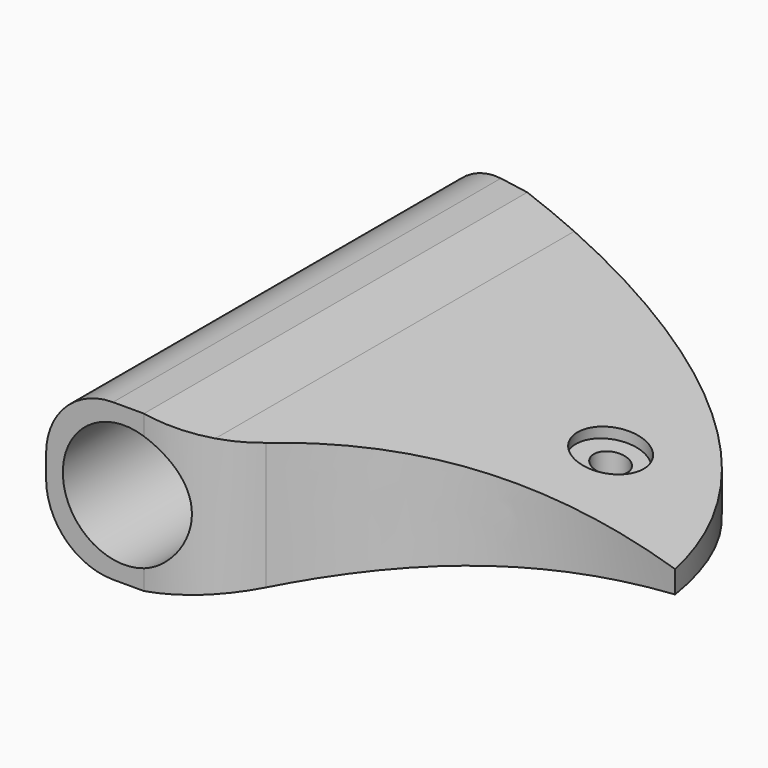
from build123d import *

# Parameters (mm, degrees)
F0_R         = 0.75
F1_DEPTH     = 7
F2_R         = 2.75
F3_DEPTH     = 25
F4_R         = 3
F6_DEPTH     = 25
F7_R         = 1.5
F8_DEPTH     = 0.5
F9_R         = 1.5
F10_DEPTH    = 0.5
F11_T4_DEPTH = 19.1627380087


# Not quite as in the source:
# - a fillet or chamfer that OpenCascade refuses, or shapes differently, is made with other operations: its cross-section is extruded or revolved along the edge and cut away or added


with BuildPart() as f1:
    # F0 (on Top) → F1 (new body)
    with BuildSketch(Plane.XY):
        with BuildLine():
            add(Edge.make_bspline(
                [(0, 11), (5.2254716866, 10.975911282), (20.5224081874, 7.3522534221), (22.6636249572, -4.0898798034)],
                knots=[0, 0, 0, 0, 27.2276397927, 27.2276397927, 27.2276397927, 27.2276397927], degree=3))
            Line((0, 11), (0, -11))
            Line((0, -11), (7, -11))
            add(Edge.make_bspline(
                [(7, -11), (10.2693928853, -5.7117650285), (14.8583007976, -2.8734656516), (22.6636249572, -4.0898798034)],
                knots=[0, 0, 0, 0, 17.1201316564, 17.1201316564, 17.1201316564, 17.1201316564], degree=3))
        make_face()
        with Locations((16.5, 0)):
            Circle(F0_R, mode=Mode.SUBTRACT)
    extrude(amount=F1_DEPTH)

    # F2 (on face) → F3 (cut)
    with BuildSketch(Plane.XZ.offset(11)):
        with Locations((3.5, 3.5)):
            Circle(F2_R)
    extrude(amount=-F3_DEPTH, mode=Mode.SUBTRACT)

    # F4
    f4_edges = [f1.edges().sort_by_distance(p)[0] for p in [
        (0, 0, 0),
        (0, 0, 7),
    ]]
    fillet(f4_edges, radius=F4_R)

    # F5 (on face) → F6 (cut)
    with BuildSketch(Plane.XZ.offset(11)):
        Polygon((7, 6.5709358384), (22.6717181504, 4), (26.1740684509, 7.8573133796), (11.5607753396, 11.3733848557), (4.3845428154, 7), (7, 7), align=None)
        Polygon((26.1740684509, -0.8573133796), (22.6717181504, 3), (7, 0.4290641616), (7, 0), (4.3845428154, 0), (11.5607753396, -4.3733848557), align=None)
        Polygon((4.3845428154, 7), (7, 6.5709358384), (7, 7), align=None)
        Polygon((7, 0), (7, 0.4290641616), (4.3845428154, 0), align=None)
    extrude(amount=-F6_DEPTH, mode=Mode.SUBTRACT)

    # F7 (on face) → F8 (cut)
    with BuildSketch(Plane(origin=(1.2331564946, 0, 7.5169830107), x_dir=(0.9868095474, 0, -0.1618855065), z_dir=(0.1618855065, 0, 0.9868095474))):
        with Locations((15.4709118351, 0)):
            Circle(F7_R)
    extrude(amount=-F8_DEPTH, mode=Mode.SUBTRACT)

    # F9 (on face) → F10 (cut)
    with BuildSketch(Plane(origin=(0.1149053506, 0, -0.7004314313), x_dir=(0.9868095474, 0, 0.1618855065), z_dir=(0.1618855065, 0, -0.9868095474))):
        with Locations((16.6041103809, 0)):
            Circle(F9_R)
    extrude(amount=-F10_DEPTH, mode=Mode.SUBTRACT)

    # F11: fillet of radius 5 on 1 edges, made by hand


with BuildPart() as f11_tool2:
    # F11_s3 → F11_t4 (new body)
    with BuildSketch(Plane.XY.offset(-6.0813690043)):
        with BuildLine():
            ThreePointArc((8.3278164384, -9.0886011335), (6.5818041274, -10.4968325334), (4.3958267336, -11))
            Line((4.3958267336, -11), (4.3958267336, -11.1))
            Line((4.3958267336, -11.1), (7, -11.1))
            Line((7, -11.1), (7.0850572831, -11.0525857262))
            ThreePointArc((7.0850572831, -11.0525857262), (7.7193199568, -10.0826857854), (8.4064562325, -9.1503731561))
            Line((8.4064562325, -9.1503731561), (8.3278164384, -9.0886011335))
        make_face()
    extrude(amount=F11_T4_DEPTH)

    split(bisect_by=Plane(origin=(0.1149053506, 0, -0.7004314313), x_dir=(0, 1, 0), z_dir=(-0.1618855065, 0, 0.9868095474)), keep=Keep.TOP)

    split(bisect_by=Plane(origin=(1.2331564946, 0, 7.5169830107), x_dir=(0, 1, 0), z_dir=(-0.1618855065, 0, -0.9868095474)), keep=Keep.TOP)


with BuildPart() as f1_1:
    add(f1.part)

    # F11_t1: cut F11_tool2
    add(f11_tool2.part, mode=Mode.SUBTRACT)


solid = f1_1.part
